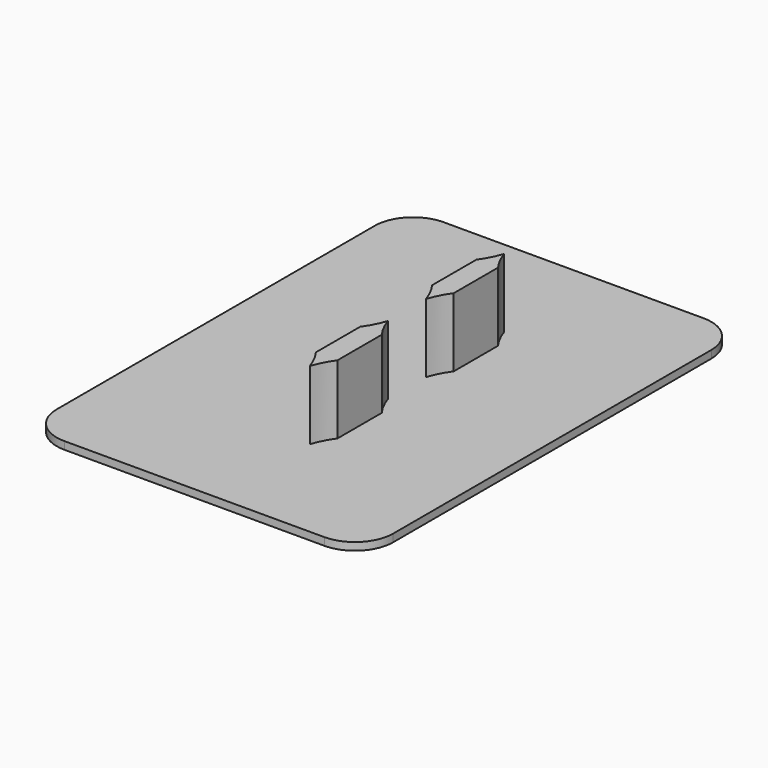
from build123d import *

# Parameters (mm, degrees)
F0_W     = 6
F0_H     = 62
F0_W_2   = 38
F1_DEPTH = 1
F2_DEPTH = 10
F3_R     = 5


# Not quite as in the source:
# - a feature names something its author has since deleted; it is built from what else it names


with BuildPart() as f1:
    # F0 (on Top) → F1 (new body)
    with BuildSketch(Plane.XY):
        with Locations((-12.5, 19)):
            Rectangle(F0_W, F0_H)
        with Locations((9.5, 19)):
            Rectangle(F0_W_2, F0_H)
        with BuildLine():
            ThreePointArc((9.5, 15.8775010008), (10.0985618966, 14.4432029131), (10.9121369044, 13.1189736826))
            Line((10.9121369044, 13.1189736826), (10.9121369044, 5.8810263174))
            ThreePointArc((10.9121369044, 5.8810263174), (10.0985618966, 4.5567970869), (9.5, 3.1224989992))
            ThreePointArc((9.5, 3.1224989992), (8.9014381034, 4.5567970869), (8.0878630956, 5.8810263174))
            Line((8.0878630956, 5.8810263174), (8.0878630956, 13.1189736826))
            ThreePointArc((8.0878630956, 13.1189736826), (8.9014381034, 14.4432029131), (9.5, 15.8775010008))
        make_face(mode=Mode.SUBTRACT)
        with BuildLine():
            Line((8.0878630956, 24.8810263174), (8.0878630956, 32.1189736826))
            ThreePointArc((8.0878630956, 32.1189736826), (8.9014381034, 33.4432029131), (9.5, 34.8775010008))
            ThreePointArc((9.5, 34.8775010008), (10.0985618966, 33.4432029131), (10.9121369044, 32.1189736826))
            Line((10.9121369044, 32.1189736826), (10.9121369044, 24.8810263174))
            ThreePointArc((10.9121369044, 24.8810263174), (10.0985618966, 23.5567970869), (9.5, 22.1224989992))
            ThreePointArc((9.5, 22.1224989992), (8.9014381034, 23.5567970869), (8.0878630956, 24.8810263174))
        make_face(mode=Mode.SUBTRACT)
    extrude(amount=F1_DEPTH)

    # F0 (on Top) → F2 (join)
    with BuildSketch(Plane.XY):
        with BuildLine():
            ThreePointArc((9.5, 34.8775010008), (8.9014381034, 33.4432029131), (8.0878630956, 32.1189736826))
            Line((8.0878630956, 32.1189736826), (8.0878630956, 24.8810263174))
            ThreePointArc((8.0878630956, 24.8810263174), (8.9014381034, 23.5567970869), (9.5, 22.1224989992))
            ThreePointArc((9.5, 22.1224989992), (10.0985618966, 23.5567970869), (10.9121369044, 24.8810263174))
            Line((10.9121369044, 24.8810263174), (10.9121369044, 32.1189736826))
            ThreePointArc((10.9121369044, 32.1189736826), (10.0985618966, 33.4432029131), (9.5, 34.8775010008))
        make_face()
        with BuildLine():
            Line((10.9121369044, 5.8810263174), (10.9121369044, 13.1189736826))
            ThreePointArc((10.9121369044, 13.1189736826), (10.0985618966, 14.4432029131), (9.5, 15.8775010008))
            ThreePointArc((9.5, 15.8775010008), (8.9014381034, 14.4432029131), (8.0878630956, 13.1189736826))
            Line((8.0878630956, 13.1189736826), (8.0878630956, 5.8810263174))
            ThreePointArc((8.0878630956, 5.8810263174), (8.9014381034, 4.5567970869), (9.5, 3.1224989992))
            ThreePointArc((9.5, 3.1224989992), (10.0985618966, 4.5567970869), (10.9121369044, 5.8810263174))
        make_face()
    extrude(amount=F2_DEPTH)

    # F3
    f3_edges = [f1.edges().sort_by_distance(p)[0] for p in [
        (-15.5, 50, 0.5),
        (28.5, 50, 0.5),
        (28.5, -12, 0.5),
        (-15.5, -12, 0.5),
    ]]
    fillet(f3_edges, radius=F3_R)


solid = f1.part
